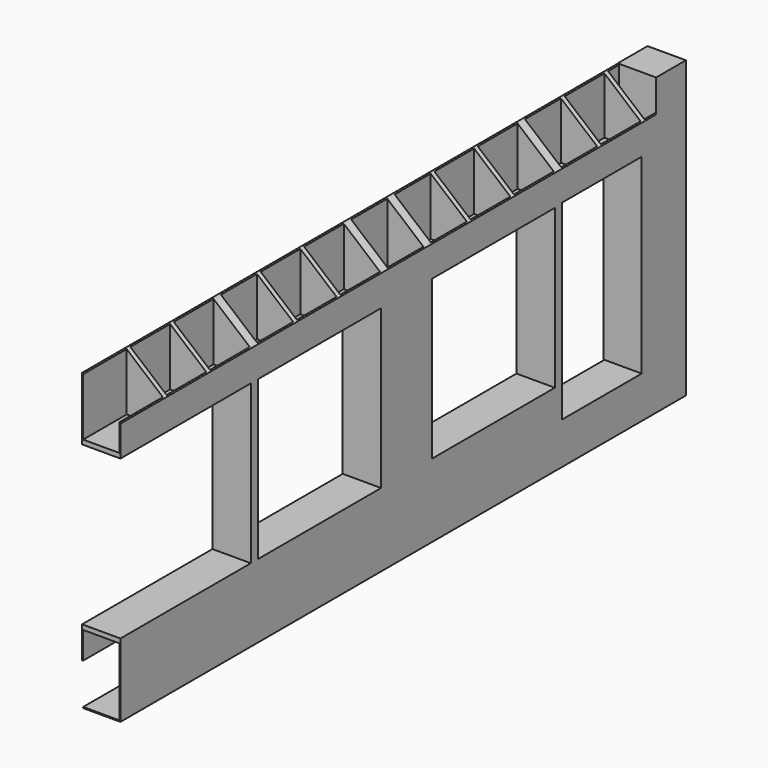
from build123d import *

# Parameters (mm, degrees)
F0_W     = 51
F0_H     = 649
F0_H_2   = 749
F0_H_3   = 3250
F1_DEPTH = 400
F0_H_4   = 399
F0_H_5   = 639
F0_H_6   = 51
F0_H_7   = 1750
F0_W_2   = 412
F2_W     = 601
F2_H     = 749
F2_W_2   = 549
F2_W_3   = 498
F2_H_2   = 649
F2_W_4   = 1698
F2_H_3   = 1750
F2_W_5   = 4109
F2_H_4   = 3250
F2_W_6   = 1098
F2_H_5   = 2110
F3_DEPTH = 12
F4_W     = 549
F4_H     = 649
F4_W_2   = 498
F4_W_3   = 601
F4_H_2   = 299
F4_W_4   = 1749
F4_H_3   = 1750
F4_W_5   = 1698
F5_DEPTH = 12
F6_W     = 412
F6_H     = 7812
F7_DEPTH = 12
F9_DEPTH = 7400


# Not quite as in the source:
# - a feature names something its author has since deleted; it is built from what else it names


with BuildPart() as f1:
    # F0 (on Right) → F1 (new body)
    with BuildSketch(Plane.YZ):
        with Locations((626.5, 2925.5)):
            Rectangle(F0_W, F0_H)
        with Locations((1226.5, 374.5)):
            Rectangle(F0_W, F0_H_2)
        with Locations((3026.5, 374.5)):
            Rectangle(F0_W, F0_H_2)
        with Locations((1226.5, 2925.5)):
            Rectangle(F0_W, F0_H)
        Polygon((1801, 2550), (1801, 800), (1801, 749), (1801, 0), (1852, 0), (1852, 3250), (1801, 3250), (1801, 2601), align=None)
        with Locations((3026.5, 2925.5)):
            Rectangle(F0_W, F0_H)
        Polygon((3601, 2550), (3601, 800), (3601, 749), (3601, 0), (3652, 0), (3652, 3250), (3601, 3250), (3601, 2601), align=None)
        Polygon((0, 800), (0, 749), (601, 749), (652, 749), (1201, 749), (1252, 749), (1801, 749), (1801, 800), align=None)
        Polygon((0, 2601), (0, 2550), (1801, 2550), (1801, 2601), (1252, 2601), (1201, 2601), (652, 2601), (601, 2601), align=None)
        with Locations((626.5, 374.5)):
            Rectangle(F0_W, F0_H_2)
        Polygon((1852, 3250), (1852, 0), (1903, 0), (1903, 749), (1903, 800), (1903, 2550), (1903, 2601), (1903, 3250), align=None)
        Polygon((1903, 800), (1903, 749), (2401, 749), (2452, 749), (3001, 749), (3052, 749), (3601, 749), (3601, 800), align=None)
        with Locations((2426.5, 374.5)):
            Rectangle(F0_W, F0_H_2)
        with Locations((2426.5, 2925.5)):
            Rectangle(F0_W, F0_H)
        Polygon((2401, 2601), (1903, 2601), (1903, 2550), (3601, 2550), (3601, 2601), (3052, 2601), (3001, 2601), (2452, 2601), align=None)
        with Locations((3677.5, 1625)):
            Rectangle(F0_W, F0_H_3)
    extrude(amount=F1_DEPTH)



with BuildPart() as f1b:
    # F0 (on Right) → F1, piece 2 (new body)
    with BuildSketch(Plane.YZ):
        with Locations((4826.5, 374.5)):
            Rectangle(F0_W, F0_H_2)
        Polygon((6001, 2550), (6001, 800), (6001, 749), (6001, 0), (6052, 0), (6052, 749), (6052, 2601), (6052, 3250), (6001, 3250), (6001, 2601), align=None)
        with Locations((6626.5, 199.5)):
            Rectangle(F0_W, F0_H_4)
        with Locations((6626.5, 2930.5)):
            Rectangle(F0_W, F0_H_5)
        Polygon((4201, 3250), (4201, 0), (4252, 0), (4252, 749), (4252, 800), (4252, 2550), (4252, 2601), (4252, 3250), align=None)
        with Locations((5426.5, 2925.5)):
            Rectangle(F0_W, F0_H)
        Polygon((7201, 399), (7201, 0), (7252, 0), (7252, 3250), (7201, 3250), (7201, 2611), (7201, 2560), (7201, 450), align=None)
        with Locations((4277.5, 774.5)):
            Rectangle(F0_W, F0_H_6)
        Polygon((4303, 800), (4303, 749), (4801, 749), (4852, 749), (5401, 749), (5452, 749), (6001, 749), (6001, 800), align=None)
        Polygon((6601, 2611), (6103, 2611), (6103, 2560), (7201, 2560), (7201, 2611), (6652, 2611), align=None)
        Polygon((6103, 450), (6103, 399), (6601, 399), (6652, 399), (7201, 399), (7201, 450), align=None)
        with Locations((5426.5, 374.5)):
            Rectangle(F0_W, F0_H_2)
        Polygon((6052, 749), (6052, 0), (6103, 0), (6103, 399), (6103, 450), (6103, 2560), (6103, 2611), (6103, 3250), (6052, 3250), (6052, 2601), align=None)
        with Locations((4826.5, 2925.5)):
            Rectangle(F0_W, F0_H)
        Polygon((4801, 2601), (4303, 2601), (4303, 2550), (6001, 2550), (6001, 2601), (5452, 2601), (5401, 2601), (4852, 2601), align=None)
        with Locations((4277.5, 2925.5)):
            Rectangle(F0_W, F0_H)
        with Locations((4277.5, 1675)):
            Rectangle(F0_W, F0_H_7)
        with Locations((4277.5, 2575.5)):
            Rectangle(F0_W, F0_H_6)
        with Locations((4277.5, 374.5)):
            Rectangle(F0_W, F0_H_2)
    extrude(amount=F1_DEPTH)


with BuildPart() as f1c:
    # F0 (on Right) → F1, piece 3 (new body)
    with BuildSketch(Plane.YZ):
        with Locations((7606, 1625)):
            Rectangle(F0_W_2, F0_H_3)
    extrude(amount=F1_DEPTH)


with BuildPart() as f1_1:
    add(f1.part)

    add(f1b.part)  # F3 merges F1b

    add(f1c.part)  # F3 merges F1c
    # F2 (on face) → F3 (join)
    with BuildSketch(Plane.YZ.offset(400)):
        with Locations((300.5, 374.5)):
            Rectangle(F2_W, F2_H)
        with Locations((926.5, 374.5)):
            Rectangle(F2_W_2, F2_H)
        with Locations((1526.5, 374.5)):
            Rectangle(F2_W_2, F2_H)
        with Locations((2152, 374.5)):
            Rectangle(F2_W_3, F2_H)
        with Locations((2726.5, 374.5)):
            Rectangle(F2_W_2, F2_H)
        with Locations((3326.5, 374.5)):
            Rectangle(F2_W_2, F2_H)
        with Locations((300.5, 2925.5)):
            Rectangle(F2_W, F2_H_2)
        with Locations((926.5, 2925.5)):
            Rectangle(F2_W_2, F2_H_2)
        with Locations((1526.5, 2925.5)):
            Rectangle(F2_W_2, F2_H_2)
        with Locations((2152, 2925.5)):
            Rectangle(F2_W_3, F2_H_2)
        with Locations((2726.5, 2925.5)):
            Rectangle(F2_W_2, F2_H_2)
        with Locations((3326.5, 2925.5)):
            Rectangle(F2_W_2, F2_H_2)
        Polygon((601, 749), (601, 0), (652, 0), (652, 749), (1201, 749), (1201, 0), (1252, 0), (1252, 749), (1801, 749), (1801, 0), (1903, 0), (1903, 749), (2401, 749), (2401, 0), (2452, 0), (2452, 749), (3001, 749), (3001, 0), (3052, 0), (3052, 749), (3601, 749), (3601, 0), (3703, 0), (3703, 3250), (3601, 3250), (3601, 2601), (3052, 2601), (3052, 3250), (3001, 3250), (3001, 2601), (2452, 2601), (2452, 3250), (2401, 3250), (2401, 2601), (1903, 2601), (1903, 3250), (1801, 3250), (1801, 2601), (1252, 2601), (1252, 3250), (1201, 3250), (1201, 2601), (652, 2601), (652, 3250), (601, 3250), (601, 2601), (0, 2601), (0, 2550), (1801, 2550), (1801, 800), (0, 800), (0, 749), align=None)
        with Locations((2752, 1675)):
            Rectangle(F2_W_4, F2_H_3, mode=Mode.SUBTRACT)
        with Locations((5757.5, 1625)):
            Rectangle(F2_W_5, F2_H_4)
        with Locations((6652, 1505)):
            Rectangle(F2_W_6, F2_H_5, mode=Mode.SUBTRACT)
        with Locations((5152, 1675)):
            Rectangle(F2_W_4, F2_H_3, mode=Mode.SUBTRACT)
    extrude(amount=F3_DEPTH)

    # F4 (on face) → F5 (join)
    with BuildSketch(Plane(origin=(0, 0, 0), x_dir=(0, -1, 0), z_dir=(-1, 0, 0))):
        with Locations((-3326.5, 2925.5)):
            Rectangle(F4_W, F4_H)
        with Locations((-2726.5, 2925.5)):
            Rectangle(F4_W, F4_H)
        with Locations((-2152, 2925.5)):
            Rectangle(F4_W_2, F4_H)
        with Locations((-1526.5, 2925.5)):
            Rectangle(F4_W, F4_H)
        with Locations((-926.5, 2925.5)):
            Rectangle(F4_W, F4_H)
        with Locations((-300.5, 2925.5)):
            Rectangle(F4_W_3, F4_H)
        with Locations((-300.5, 599.5)):
            Rectangle(F4_W_3, F4_H_2)
        Polygon((-3703, 450), (-3703, 3250), (-7812, 3250), (-7812, 450), (-7201, 450), (-7201, 2560), (-6103, 2560), (-6103, 450), align=None)
        with Locations((-5126.5, 1675)):
            Rectangle(F4_W_4, F4_H_3, mode=Mode.SUBTRACT)
        with Locations((-3326.5, 599.5)):
            Rectangle(F4_W, F4_H_2)
        with Locations((-2726.5, 599.5)):
            Rectangle(F4_W, F4_H_2)
        with Locations((-2152, 599.5)):
            Rectangle(F4_W_2, F4_H_2)
        with Locations((-1526.5, 599.5)):
            Rectangle(F4_W, F4_H_2)
        with Locations((-926.5, 599.5)):
            Rectangle(F4_W, F4_H_2)
        Polygon((-1801, 800), (-1801, 2550), (0, 2550), (0, 2601), (-601, 2601), (-601, 3250), (-652, 3250), (-652, 2601), (-1201, 2601), (-1201, 3250), (-1252, 3250), (-1252, 2601), (-1801, 2601), (-1801, 3250), (-1903, 3250), (-1903, 2601), (-2401, 2601), (-2401, 3250), (-2452, 3250), (-2452, 2601), (-3001, 2601), (-3001, 3250), (-3052, 3250), (-3052, 2601), (-3601, 2601), (-3601, 3250), (-3703, 3250), (-3703, 450), (-3601, 450), (-3601, 749), (-3052, 749), (-3052, 450), (-3001, 450), (-3001, 749), (-2452, 749), (-2452, 450), (-2401, 450), (-2401, 749), (-1903, 749), (-1903, 450), (-1801, 450), (-1801, 749), (-1252, 749), (-1252, 450), (-1201, 450), (-1201, 749), (-652, 749), (-652, 450), (-601, 450), (-601, 749), (0, 749), (0, 800), align=None)
        with Locations((-2752, 1675)):
            Rectangle(F4_W_5, F4_H_3, mode=Mode.SUBTRACT)
    extrude(amount=F5_DEPTH)

    # F6 (on face) → F7 (join)
    with BuildSketch(Plane(origin=(0, 0, 0), x_dir=(1, 0, 0), z_dir=(0, 0, -1))):
        with Locations((206, -3906)):
            Rectangle(F6_W, F6_H)
    extrude(amount=F7_DEPTH)

    # F8 (on face) → F9 (cut)
    with BuildSketch(Plane.XZ):
        Polygon((0, 3237.1461581129), (400, 2900), (515.7678202297, 2802.4233104411), (515.7678202297, 3337.787177324), (-119.4034299835, 3337.787177324), (-12, 3247.2605428563), align=None)
    extrude(amount=-F9_DEPTH, mode=Mode.SUBTRACT)


solid = f1_1.part
